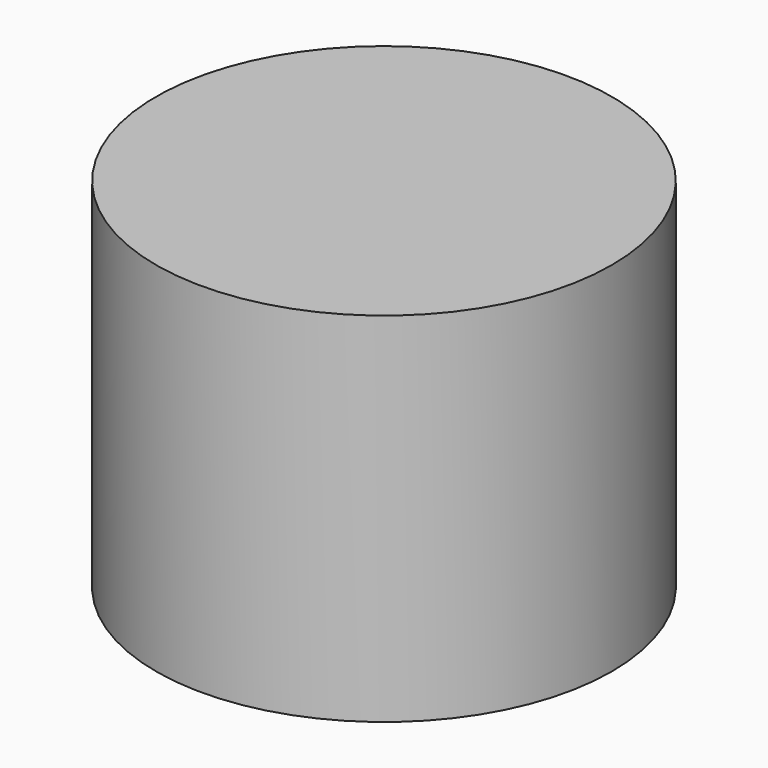
from build123d import *

# Parameters (mm, degrees)
F2_R     = 5.9863215471
F4_DEPTH = 9.398


# Not quite as in the source:
# - the program builds the solid bodies; features that only make, move or delete a surface that nothing else refers to are left out


with BuildPart() as f4:
    # F2 (on Top) → F4 (new body)
    with BuildSketch(Plane.XY):
        with Locations((-15.9957297146, 16.0671286285)):
            Circle(F2_R)
    extrude(amount=F4_DEPTH)


solid = f4.part
